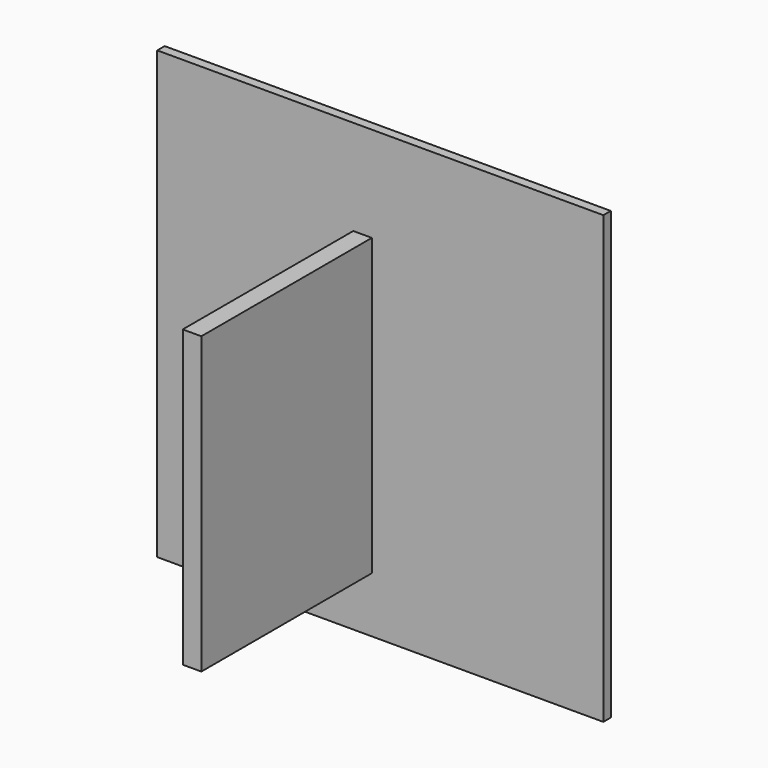
from build123d import *

# Parameters (mm, degrees)
F0_W     = 152.4
F0_H     = 152.4
F1_DEPTH = 3.175
F3_DEPTH = 6.35


# Not quite as in the source:
# - a length typed as a fraction of an inch, garbled in the dataset ("3 / 203.2 mm" for 3/8 in), is restored
# - a feature names something its author has since deleted; it is built from what else it names


with BuildPart() as f1:
    # F0 (on Front) → F1 (new body)
    with BuildSketch(Plane.XZ):
        with Locations((9.2369243503, 5.9638554769)):
            Rectangle(F0_W, F0_H)
    extrude(amount=F1_DEPTH)

    # F2 (on Right) → F3 (join)
    with BuildSketch(Plane.YZ):
        Polygon((0, 0), (0, 49.6197640896), (-75.9790167212, 49.6197640896), (-75.9790167212, -51.2280538678), (0, -51.2280538678), align=None)
    extrude(amount=F3_DEPTH)


solid = f1.part
